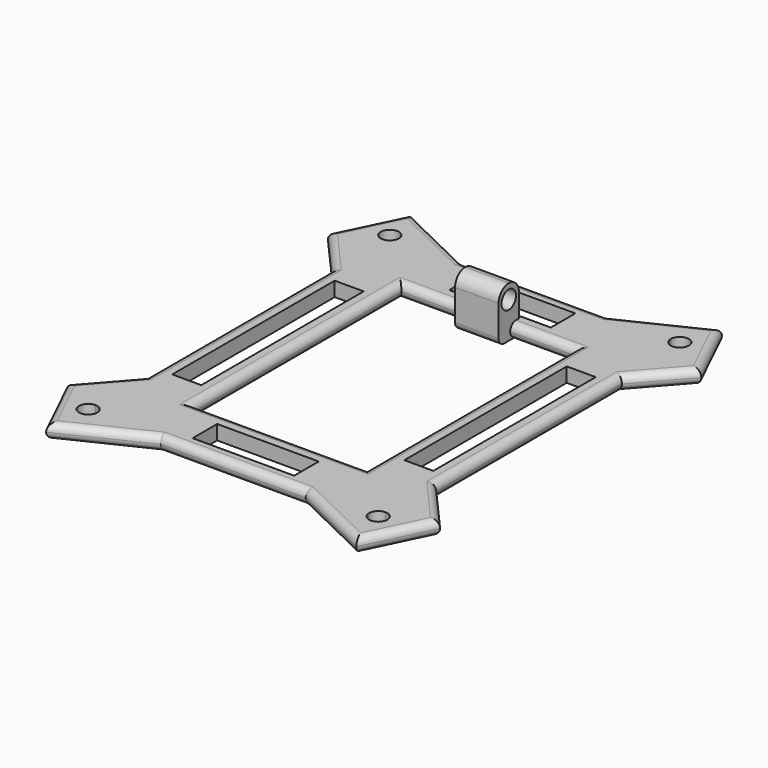
from build123d import *

# Parameters (mm, degrees)
F0_W     = 14
F0_H     = 4.2391675711
F0_W_2   = 4
F0_H_2   = 28
F1_DEPTH = 2
F0_W_3   = 6
F0_H_3   = 2
F0_H_4   = 1.5
F2_DEPTH = 7
F3_R     = 1.74999
F4_R     = 1.25
F5_DEPTH = 25
F6_R     = 0.99999


# Not quite as in the source:
# - a fillet or chamfer is up to 0.001 mm smaller than in the source, because OpenCascade refuses the exact size
# - a feature names something its author has since deleted; it is built from what else it names


with BuildPart() as f1:
    # F0 (on Top) → F1 (new body)
    with BuildSketch(Plane.XY):
        with BuildLine():
            Line((-10, -26), (10, -26))
            ThreePointArc((10, -26), (12.9289321881, -18.9289321881), (20, -16))
            Line((20, -16), (20, 16))
            ThreePointArc((20, 16), (12.9289321881, 18.9289321881), (10, 26))
            Line((10, 26), (-10, 26))
            ThreePointArc((-10, 26), (-12.9289321881, 18.9289321881), (-20, 16))
            Line((-20, 16), (-20, -16))
            ThreePointArc((-20, -16), (-12.9289321881, -18.9289321881), (-10, -26))
        make_face()
        with Locations((0, -22.1195837855)):
            Rectangle(F0_W, F0_H, mode=Mode.SUBTRACT)
        with Locations((-16, 0)):
            Rectangle(F0_W_2, F0_H_2, mode=Mode.SUBTRACT)
        Polygon((3, 18), (10, 18), (12, 18), (12, -18), (-12, -18), (-12, 18), (-10, 18), (-3, 18), (-3, 19.5), (3, 19.5), align=None, mode=Mode.SUBTRACT)
        with Locations((16, 0)):
            Rectangle(F0_W_2, F0_H_2, mode=Mode.SUBTRACT)
        with Locations((0, 22.1195837855)):
            Rectangle(F0_W, F0_H, mode=Mode.SUBTRACT)
        with BuildLine():
            Line((-20, 24.75), (-20, 16))
            ThreePointArc((-20, 16), (-12.9289321881, 18.9289321881), (-10, 26))
            Line((-10, 26), (-18.75, 26))
            ThreePointArc((-18.75, 26), (-19.1161165235, 25.1161165235), (-20, 24.75))
        make_face()
        with BuildLine():
            Line((-25.7454968465, 22.5147810633), (-20, 16))
            Line((-20, 16), (-20, 24.75))
            ThreePointArc((-20, 24.75), (-20.8838834765, 26.8838834765), (-18.75, 26))
            Line((-18.75, 26), (-10, 26))
            Line((-10, 26), (-21.386597903, 31.5147810633))
            Line((-21.386597903, 31.5147810633), (-25.7454968465, 22.5147810633))
        make_face()
        with BuildLine():
            ThreePointArc((10, 26), (12.9289321881, 18.9289321881), (20, 16))
            Line((20, 16), (20, 24.75))
            ThreePointArc((20, 24.75), (19.1161165235, 25.1161165235), (18.75, 26))
            Line((18.75, 26), (10, 26))
        make_face()
        with BuildLine():
            Line((20, 24.75), (20, 16))
            Line((20, 16), (25.7454968465, 22.5147810633))
            Line((25.7454968465, 22.5147810633), (21.386597903, 31.5147810633))
            Line((21.386597903, 31.5147810633), (10, 26))
            Line((10, 26), (18.75, 26))
            ThreePointArc((18.75, 26), (20, 27.25), (21.25, 26))
            ThreePointArc((21.25, 26), (20.8838834765, 25.1161165235), (20, 24.75))
        make_face()
        with BuildLine():
            ThreePointArc((20, -16), (12.9289321881, -18.9289321881), (10, -26))
            Line((10, -26), (18.75, -26))
            ThreePointArc((18.75, -26), (19.1161165235, -25.1161165235), (20, -24.75))
            Line((20, -24.75), (20, -16))
        make_face()
        with BuildLine():
            Line((18.75, -26), (10, -26))
            Line((10, -26), (21.386597903, -31.5147810633))
            Line((21.386597903, -31.5147810633), (25.7454968465, -22.5147810633))
            Line((25.7454968465, -22.5147810633), (20, -16))
            Line((20, -16), (20, -24.75))
            ThreePointArc((20, -24.75), (20.8838834765, -25.1161165235), (21.25, -26))
            ThreePointArc((21.25, -26), (20, -27.25), (18.75, -26))
        make_face()
        with BuildLine():
            Line((-21.386597903, -31.5147810633), (-10, -26))
            Line((-10, -26), (-18.75, -26))
            ThreePointArc((-18.75, -26), (-20.8838834765, -26.8838834765), (-20, -24.75))
            Line((-20, -24.75), (-20, -16))
            Line((-20, -16), (-25.7454968465, -22.5147810633))
            Line((-25.7454968465, -22.5147810633), (-21.386597903, -31.5147810633))
        make_face()
        with BuildLine():
            Line((-18.75, -26), (-10, -26))
            ThreePointArc((-10, -26), (-12.9289321881, -18.9289321881), (-20, -16))
            Line((-20, -16), (-20, -24.75))
            ThreePointArc((-20, -24.75), (-19.1161165235, -25.1161165235), (-18.75, -26))
        make_face()
    extrude(amount=F1_DEPTH)

    # F0 (on Top) → F2 (join)
    with BuildSketch(Plane.XY):
        with Locations((0, 17)):
            Rectangle(F0_W_3, F0_H_3)
        with Locations((0, 18.75)):
            Rectangle(F0_W_3, F0_H_4)
    extrude(amount=F2_DEPTH)

    # F3 (radius 1.75 in the source; OpenCascade refuses exactly that, so slightly less here)
    f3_edges = [f1.edges().sort_by_distance(p)[0] for p in [
        (0, 16, 7),
        (0, 19.5, 7),
    ]]
    fillet(f3_edges, radius=F3_R)

    # F4 (on face) → F5 (cut)
    with BuildSketch(Plane(origin=(-3, 0, 0), x_dir=(0, -1, 0), z_dir=(-1, 0, 0))):
        with Locations((-17.75, 5)):
            Circle(F4_R)
    extrude(amount=-F5_DEPTH, mode=Mode.SUBTRACT)

    # F6 (radius 1 in the source; OpenCascade refuses exactly that, so slightly less here)
    f6_edges = [f1.edges().sort_by_distance(p)[0] for p in [
        (-20, 0, 2),
        (-23.566047, -27.014781, 2),
        (0, -26, 2),
        (20, 0, 2),
        (15.693299, 28.757391, 2),
        (0, 26, 2),
        (-23.566047, 27.014781, 2),
        (-23.566047, 27.014781, 0),
        (0, 26, 0),
        (15.693299, 28.757391, 0),
        (20, 0, 0),
        (-23.566047, -27.014781, 0),
        (0, -26, 0),
        (-20, 0, 0),
        (-12, 0, 2),
        (-7.5, 18, 2),
        (7.5, 18, 2),
        (12, 0, 2),
        (0, -18, 2),
        (0, 16, 0),
        (-12, 0, 0),
        (0, -18, 0),
        (12, 0, 0),
        (-22.872748, 19.257391, 2),
        (-22.872748, 19.257391, 0),
        (-15.693299, 28.757391, 2),
        (-15.693299, 28.757391, 0),
        (22.872748, 19.257391, 2),
        (22.872748, 19.257391, 0),
        (22.872748, -19.257391, 2),
        (22.872748, -19.257391, 0),
        (15.693299, -28.757391, 0),
        (15.693299, -28.757391, 2),
        (-15.693299, -28.757391, 0),
        (-15.693299, -28.757391, 2),
        (-22.872748, -19.257391, 0),
        (-22.872748, -19.257391, 2),
        (7.5, 18, 0),
        (-7.5, 18, 0),
        (23.566047, -27.014781, 2),
        (23.566047, -27.014781, 0),
        (23.566047, 27.014781, 2),
        (23.566047, 27.014781, 0),
    ]]
    fillet(f6_edges, radius=F6_R)


solid = f1.part
